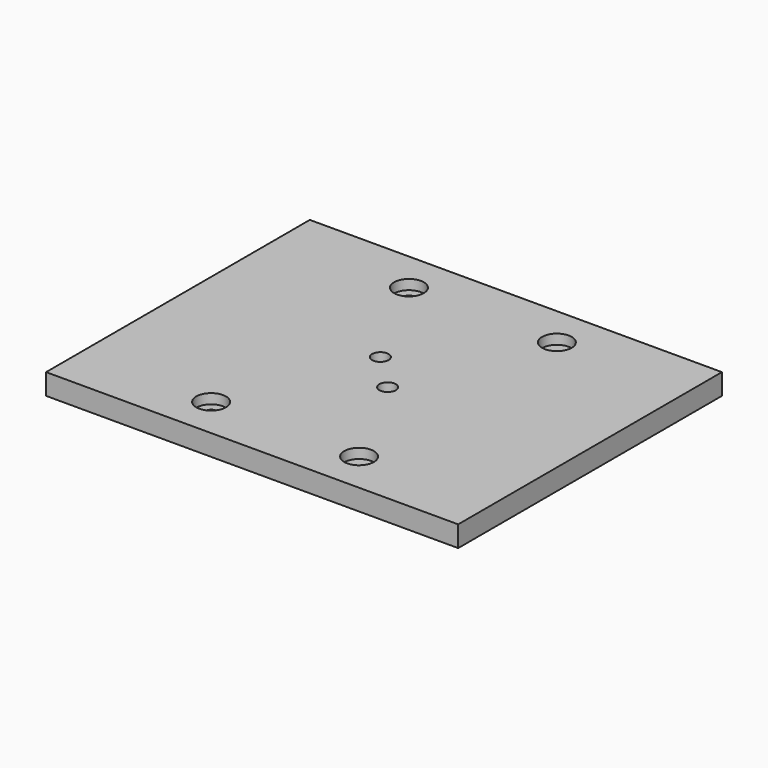
from build123d import *

# Parameters (mm, degrees)
F0_W     = 250
F0_H     = 200
F0_R     = 3.56
F0_R_2   = 2.5
F1_DEPTH = 12.7
F2_R     = 9
F2_R_2   = 5
F3_DEPTH = 6


# Not quite as in the source:
# - a length typed as a fraction of an inch, garbled in the dataset ("3 / 203.2 mm" for 3/8 in), is restored


with BuildPart() as f1:
    # F0 (on Top) → F1 (new body)
    with BuildSketch(Plane.XY):
        Rectangle(F0_W, F0_H)
        with Locations((-44.875, -75)):
            Circle(F0_R, mode=Mode.SUBTRACT)
        with Locations((44.875, -75)):
            Circle(F0_R_2, mode=Mode.SUBTRACT)
        with Locations((11, -11)):
            Circle(F0_R_2, mode=Mode.SUBTRACT)
        with Locations((-11, 11)):
            Circle(F0_R_2, mode=Mode.SUBTRACT)
        with Locations((-44.875, 75)):
            Circle(F0_R, mode=Mode.SUBTRACT)
        with Locations((44.875, 75)):
            Circle(F0_R_2, mode=Mode.SUBTRACT)
    extrude(amount=F1_DEPTH)

    # F2 (on face) → F3 (cut)
    with BuildSketch(Plane.XY.offset(12.7)):
        with Locations((-44.875, 75)):
            Circle(F2_R)
        with Locations((44.875, 75)):
            Circle(F2_R)
        with Locations((-44.875, -75)):
            Circle(F2_R)
        with Locations((44.875, -75)):
            Circle(F2_R)
        with Locations((-11, 11)):
            Circle(F2_R_2)
        with Locations((11, -11)):
            Circle(F2_R_2)
    extrude(amount=-F3_DEPTH, mode=Mode.SUBTRACT)


solid = f1.part
